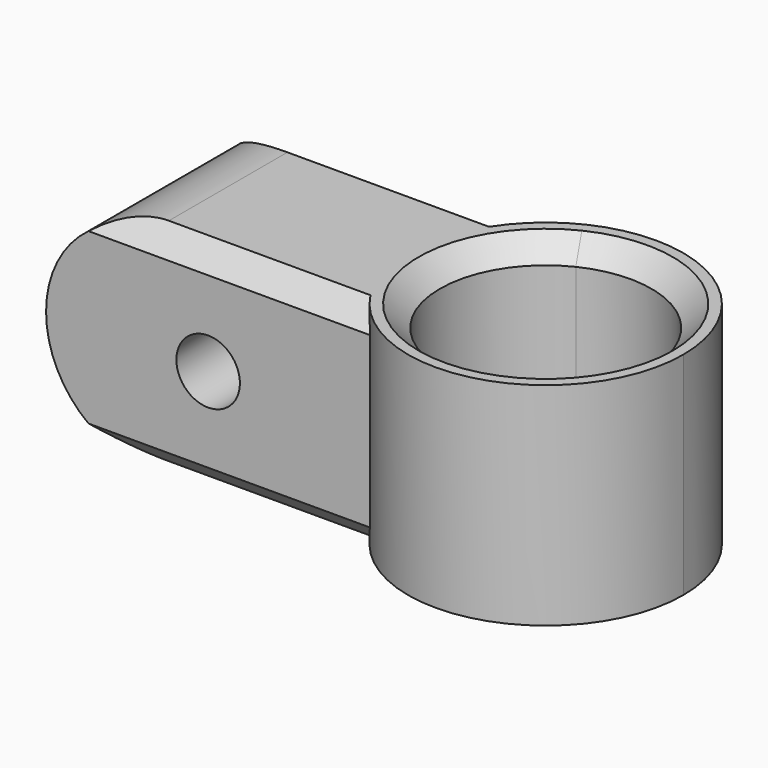
from build123d import *

# Parameters (mm, degrees)
F1_DEPTH = 10
F3_D     = 3
F3_DEPTH = 30
F3_TIP   = 0.9012909285
F4_SIZE  = 1
F5_R     = 4.99999


# Not quite as in the source:
# - a fillet or chamfer is up to 0.001 mm smaller than in the source, because OpenCascade refuses the exact size


with BuildPart() as f1:
    # F0 (on Top) → F1 (new body)
    with BuildSketch(Plane.XY):
        with BuildLine():
            Line((5.3095842402, 4.5), (-10, 4.5))
            Line((-10, 4.5), (-10, -4.5))
            Line((-10, -4.5), (5.3095842402, -4.5))
            ThreePointArc((5.3095842402, -4.5), (3.5, 0), (5.3095842402, 4.5))
        make_face()
        with BuildLine():
            Line((7.8205505282, 4.5), (5.3095842402, 4.5))
            ThreePointArc((5.3095842402, 4.5), (3.5, 0), (5.3095842402, -4.5))
            Line((5.3095842402, -4.5), (7.8205505282, -4.5))
            ThreePointArc((7.8205505282, -4.5), (5, 0), (7.8205505282, 4.5))
        make_face()
        with BuildLine():
            ThreePointArc((16.5, 0), (12.4251079936, 6.0306592691), (5.3095842402, 4.5))
            Line((5.3095842402, 4.5), (7.8205505282, 4.5))
            ThreePointArc((7.8205505282, 4.5), (12.655442773, 4.2365816031), (15, 0))
            ThreePointArc((15, 0), (12.655442773, -4.2365816031), (7.8205505282, -4.5))
            Line((7.8205505282, -4.5), (5.3095842402, -4.5))
            ThreePointArc((5.3095842402, -4.5), (12.4251079936, -6.0306592691), (16.5, 0))
        make_face()
    extrude(amount=F1_DEPTH)

    # F3
    with Locations(Plane.XZ.offset(4.5)):
        with Locations((-2.3452078799, 5)):
            Hole(F3_D / 2, depth=F3_DEPTH)
            with Locations((0, 0, -(F3_DEPTH + F3_TIP / 2))):  # 118° drill point
                Cone(0, F3_D / 2, F3_TIP, mode=Mode.SUBTRACT)

    # F4
    f4_edges = [f1.edges().sort_by_distance(p)[0] for p in [
        (12.179449, -4.5, 10),
        (12.179449, -4.5, 0),
        (-2.345208, 4.5, 10),
        (-2.345208, -4.5, 10),
        (-2.345208, -4.5, 0),
        (-2.345208, 4.5, 0),
    ]]
    chamfer(f4_edges, length=F4_SIZE)

    # F5 (radius 5 in the source; OpenCascade refuses exactly that, so slightly less here)
    f5_edges = [f1.edges().sort_by_distance(p)[0] for p in [
        (-10, 0, 10),
        (-10, 0, 0),
    ]]
    fillet(f5_edges, radius=F5_R)


solid = f1.part
